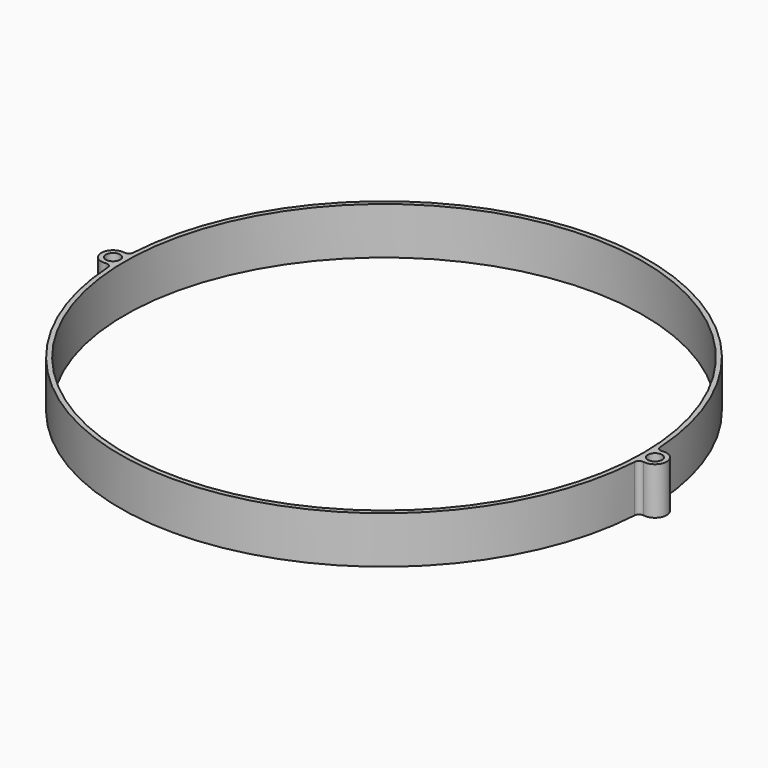
from build123d import *

# Parameters (mm, degrees)
F0_W     = 1
F0_H     = 10
F2_R     = 1.5
F3_DEPTH = 10


# Not quite as in the source:
# - a pattern or mirror of a feature is missing from the dataset's text; its kind, count and spacing are read off the source's solid


with BuildPart() as f1:
    # F0 (on Front) → F1 (revolve)
    with BuildSketch(Plane.XZ):
        with Locations((55.5, 5)):
            Rectangle(F0_W, F0_H)
    revolve(axis=Axis((0, 0, 25.0742025673), (0, 0, 1)))

    # F2 (on Top) → F3 (join)
    with BuildSketch(Plane.XY):
        with BuildLine():
            ThreePointArc((55.8974828375, -3.3869473613), (56.2759455722, -2.6625949972), (57.0683229814, -2.4624489744))
            ThreePointArc((57.0683229814, -2.4624489744), (60, 0), (57.0683229814, 2.4624489744))
            ThreePointArc((57.0683229814, 2.4624489744), (56.2759455722, 2.6625949972), (55.8974828375, 3.3869473613))
            Line((55.8974828375, 3.3869473613), (55.3983981693, 3.3567067599))
            ThreePointArc((55.3983981693, 3.3567067599), (55.5, 0), (55.3983981693, -3.3567067599))
            Line((55.3983981693, -3.3567067599), (55.8974828375, -3.3869473613))
        make_face()
        with Locations((57.5, 0)):
            Circle(F2_R, mode=Mode.SUBTRACT)
    f3 = extrude(amount=F3_DEPTH)

    # F3_copies: F3 across plane
    add(f3.mirror(Plane(origin=(0, 0, 0), x_dir=(0, 0, -1), z_dir=(-1, 0, 0))))


solid = f1.part
